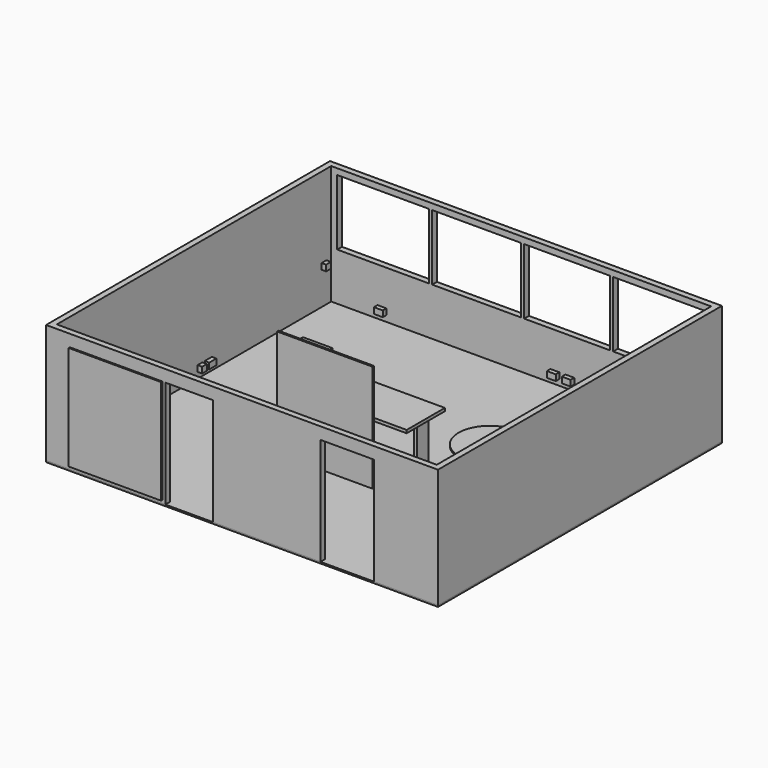
from build123d import *

# Parameters (mm, degrees)
F0_W      = 6570
F0_H      = 5950
F0_W_2    = 6370
F0_H_2    = 5750
F1_DEPTH  = 2000
F2_DEPTH  = 25
F3_W      = 800
F3_H      = 1800
F3_W_2    = 900
F3_W_3    = 1550
F3_H_2    = 1750
F4_DEPTH  = 100
F5_DEPTH  = 25
F6_W      = 1542.5
F6_H      = 1100
F6_W_2    = 1492.5
F6_W_3    = 1442.5
F7_DEPTH  = 100
F9_DEPTH  = 650
F10_W     = 1400
F10_H     = 800
F10_W_2   = 50
F10_H_2   = 250
F11_DEPTH = 50
F8_W      = 50
F8_H      = 250
F12_DEPTH = 650
F8_R      = 250
F13_DEPTH = 25
F14_R     = 525
F14_W     = 50
F14_H     = 250
F15_DEPTH = 25
F16_W     = 100
F16_H     = 100
F16_W_2   = 150
F17_DEPTH = 75
F18_W     = 150
F18_H     = 100
F18_W_2   = 100
F19_DEPTH = 75
F20_W     = 150
F20_H     = 100
F21_DEPTH = 75
F22_W     = 150
F22_H     = 100
F22_W_2   = 100
F23_DEPTH = 75
F24_W     = 500
F24_H     = 500
F25_DEPTH = 800
F26_W     = 500
F26_H     = 250
F27_DEPTH = 270
F28_W     = 1600
F28_H     = 30
F29_DEPTH = 1800


with BuildPart() as f1:
    # F0 (on Top) → F1 (new body)
    with BuildSketch(Plane.XY):
        Rectangle(F0_W, F0_H)
        Rectangle(F0_W_2, F0_H_2, mode=Mode.SUBTRACT)
    extrude(amount=F1_DEPTH)

    # F3 (on face) → F4 (cut, through all)
    with BuildSketch(Plane.XZ.offset(2975)):
        with Locations((-885, 900)):
            Rectangle(F3_W, F3_H)
        with Locations((1765, 900)):
            Rectangle(F3_W_2, F3_H)
        with Locations((-2110, 925)):
            Rectangle(F3_W_3, F3_H_2)
    extrude(amount=-F4_DEPTH, mode=Mode.SUBTRACT)

    # F6 (on face) → F7 (cut, through all)
    with BuildSketch(Plane.XZ.offset(-2875)):
        with Locations((-2313.75, 1350)):
            Rectangle(F6_W, F6_H)
        with Locations((-746.25, 1350)):
            Rectangle(F6_W_2, F6_H)
        with Locations((771.25, 1350)):
            Rectangle(F6_W_3, F6_H)
        with Locations((2313.75, 1350)):
            Rectangle(F6_W, F6_H)
    extrude(amount=-F7_DEPTH, mode=Mode.SUBTRACT)

    # F16 (on face) → F17 (join)
    with BuildSketch(Plane.YZ.offset(-3185)):
        with Locations((2725, 600)):
            Rectangle(F16_W, F16_H)
        with Locations((125, 150)):
            Rectangle(F16_W, F16_H)
        with Locations((300, 150)):
            Rectangle(F16_W_2, F16_H)
        with Locations((-1925, 150)):
            Rectangle(F16_W, F16_H)
    extrude(amount=F17_DEPTH)

    # F18 (on face) → F19 (join)
    with BuildSketch(Plane(origin=(0, -2875, 0), x_dir=(-1, 0, 0), z_dir=(0, 1, 0))):
        with Locations((3010, 150)):
            Rectangle(F18_W, F18_H)
        with Locations((-390, 150)):
            Rectangle(F18_W, F18_H)
        with Locations((-1165, 150)):
            Rectangle(F18_W_2, F18_H)
    extrude(amount=F19_DEPTH)

    # F20 (on face) → F21 (join)
    with BuildSketch(Plane(origin=(3185, 0, 0), x_dir=(0, -1, 0), z_dir=(-1, 0, 0))):
        with Locations((-550, 150)):
            Rectangle(F20_W, F20_H)
    extrude(amount=F21_DEPTH)

    # F22 (on face) → F23 (join)
    with BuildSketch(Plane.XZ.offset(-2875)):
        with Locations((-2335, 150)):
            Rectangle(F22_W, F22_H)
        with Locations((565, 150)):
            Rectangle(F22_W, F22_H)
        with Locations((815, 150)):
            Rectangle(F22_W, F22_H)
        with Locations((2915, 150)):
            Rectangle(F22_W_2, F22_H)
    extrude(amount=F23_DEPTH)


with BuildPart() as f2:
    # F0 (on Top) → F2 (new body)
    with BuildSketch(Plane.XY):
        Rectangle(F0_W, F0_H)
        Rectangle(F0_W_2, F0_H_2, mode=Mode.SUBTRACT)
        Rectangle(F0_W_2, F0_H_2)
    extrude(amount=-F2_DEPTH)


with BuildPart() as f5:
    # F3 (on face) → F5 (new body)
    with BuildSketch(Plane.XZ.offset(2975)):
        with Locations((-2110, 925)):
            Rectangle(F3_W_3, F3_H_2)
    extrude(amount=F5_DEPTH)


with BuildPart() as f9:
    # F8 (on Top) → F9 (new body)
    with BuildSketch(Plane.XY):
        Polygon((-600, 2.5), (-600, 125), (-650, 125), (-650, -125), (-600, -125), (-600, -2.5), align=None)
    extrude(amount=F9_DEPTH)



with BuildPart() as f9b:
    # F8 (on Top) → F9, piece 2 (new body)
    with BuildSketch(Plane.XY):
        Polygon((600, 125), (600, 2.5), (600, -2.5), (600, -125), (650, -125), (650, 125), align=None)
    extrude(amount=F9_DEPTH)


with BuildPart() as f9_1:
    add(f9.part)

    add(f9b.part)  # F11 merges F9b
    # F10 (on face) → F11 (join)
    with BuildSketch(Plane.XY.offset(650)):
        Rectangle(F10_W, F10_H)
        with Locations((-625, 0)):
            Rectangle(F10_W_2, F10_H_2, mode=Mode.SUBTRACT)
        with Locations((-625, 0)):
            Rectangle(F10_W_2, F10_H_2)
    extrude(amount=F11_DEPTH)


with BuildPart() as f12:
    # F8 (on Top) → F12 (new body)
    with BuildSketch(Plane.XY):
        with Locations((1775, 0)):
            Rectangle(F8_W, F8_H)
    extrude(amount=F12_DEPTH)

    # F8 (on Top) → F13 (join)
    with BuildSketch(Plane.XY):
        with Locations((1775, 0)):
            Circle(F8_R)
        with Locations((1775, 0)):
            Rectangle(F8_W, F8_H, mode=Mode.SUBTRACT)
    extrude(amount=F13_DEPTH)

    # F14 (on face) → F15 (join)
    with BuildSketch(Plane.XY.offset(650)):
        with Locations((1775, 0)):
            Circle(F14_R)
        with Locations((1775, 0)):
            Rectangle(F14_W, F14_H, mode=Mode.SUBTRACT)
        with Locations((1775, 0)):
            Rectangle(F14_W, F14_H)
    extrude(amount=F15_DEPTH)


with BuildPart() as f25:
    # F24 (on face) → F25 (new body)
    with BuildSketch(Plane.XY):
        with Locations((-1309.2528581619, 0)):
            Rectangle(F24_W, F24_H)
    extrude(amount=F25_DEPTH)

    # F26 (on face) → F27 (join)
    with BuildSketch(Plane.XY.offset(800)):
        with Locations((-1309.2528581619, 125)):
            Rectangle(F26_W, F26_H)
    extrude(amount=F27_DEPTH)


with BuildPart() as f29:
    # F28 (on face) → F29 (new body)
    with BuildSketch(Plane.XY):
        with Locations((-248.1821009796, -915.4608845711)):
            Rectangle(F28_W, F28_H)
    extrude(amount=F29_DEPTH)


solid = Compound([f1.part, f2.part, f5.part, f9_1.part, f12.part, f25.part, f29.part])
